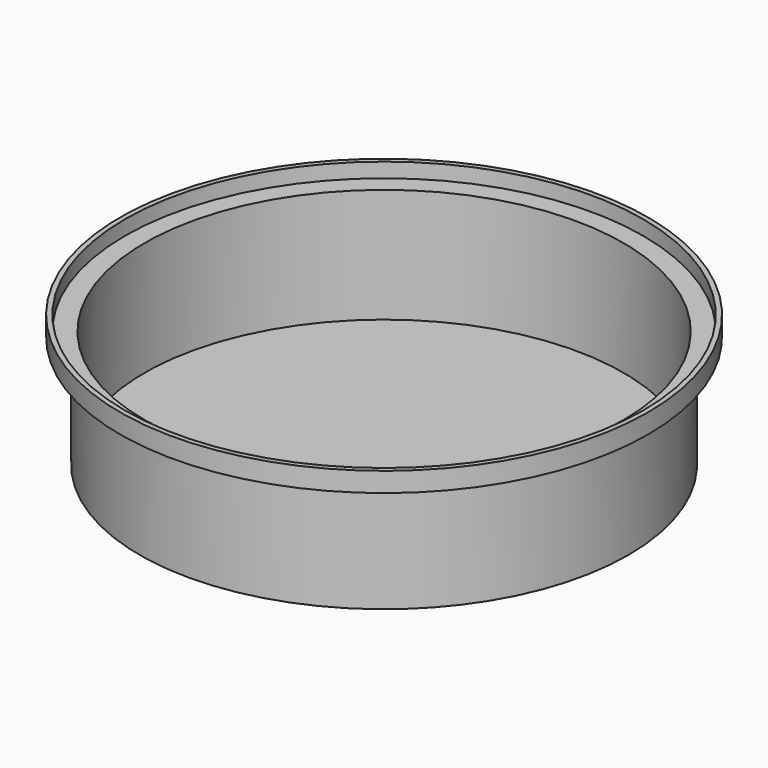
from build123d import *

# Parameters (mm, degrees)
F2_T     = -1.27
F3_R     = 62.23
F4_DEPTH = 0.47


with BuildPart() as f1:
    # F0 (on Front) → F1 (revolve)
    with BuildSketch(Plane.XZ):
        Polygon((0, 34.29), (0, 0), (63.5, 0), (63.5, 29.21), (68.58, 29.21), (68.58, 34.29), align=None)
    revolve(axis=Axis((0, 0, -14.2717824864), (0, 0, -1)))

    # F2
    f2_openings = [f1.faces().sort_by_distance(p)[0] for p in [
        (0, 0, 34.29),
    ]]
    offset(amount=F2_T, openings=f2_openings, kind=Kind.INTERSECTION)

    # F3 (on face) → F4 (cut, through all)
    with BuildSketch(Plane.XY.offset(1.27)):
        Circle(F3_R)
    extrude(amount=-F4_DEPTH, mode=Mode.SUBTRACT)


solid = f1.part
